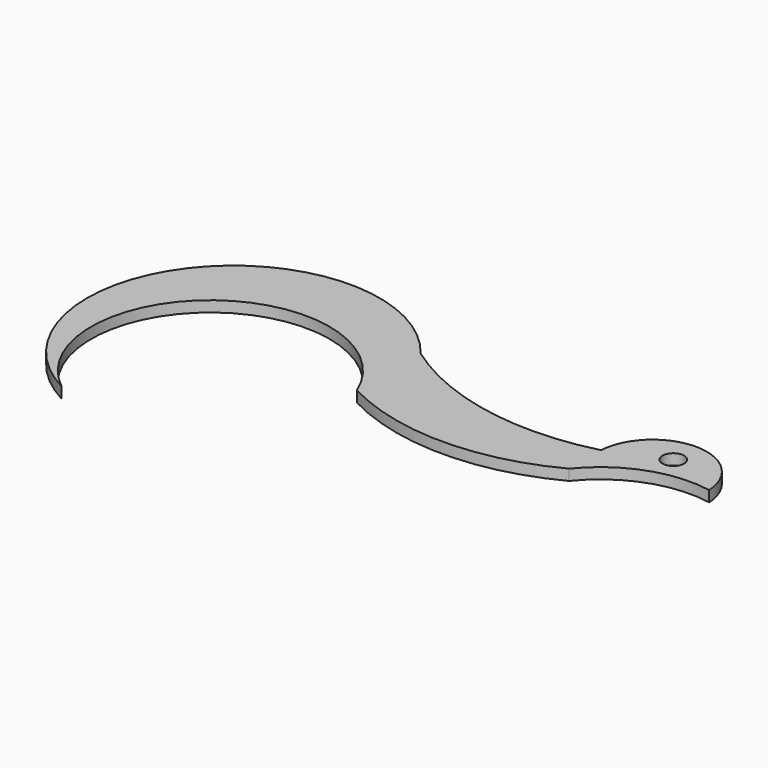
from build123d import *

# Parameters (mm, degrees)
F1_DEPTH = 5
F2_R     = 5
F3_DEPTH = 389
F4_R     = 5
F5_DEPTH = 5.001


# Not quite as in the source:
# - an extrude ends at something that could not be found from the text; its depth is read off the source's solid


with BuildPart() as f1:
    # F0 (on Top) → F1 (new body)
    with BuildSketch(Plane.XY):
        with BuildLine():
            ThreePointArc((182.6944426466, 42.1886855807), (131.7434290728, 40.4795108007), (84.8448510232, 60.4657670673))
            ThreePointArc((84.8448510232, 60.4657670673), (-20.2682643936, 62.6366103984), (0, -40.5267409035))
            ThreePointArc((0, -40.5267409035), (0.8188047448, 46.5454009095), (84.8448510232, 23.7013236039))
            ThreePointArc((84.8448510232, 23.7013236039), (133.7696468349, 11.680757797), (182.6944426466, 23.7013236039))
            ThreePointArc((182.6944426466, 23.7013236039), (205.0971207079, 39.8391466865), (232.6069186924, 42.1886855807))
            ThreePointArc((232.6069186924, 42.1886855807), (207.6506806695, 65.7101106777), (182.6944426466, 42.1886855807))
        make_face()
    extrude(amount=F1_DEPTH)

    # F2 (on Top) → F3 (cut, through all)
    with BuildSketch(Plane.XY):
        with Locations((210.5412267722, 54.1418395773)):
            Circle(F2_R)
    extrude(amount=-F3_DEPTH, mode=Mode.SUBTRACT)

    # F4 (on face) → F5 (cut, through all)
    with BuildSketch(Plane.XY.offset(5)):
        with Locations((207.6506806695, 52.6958927512)):
            Circle(F4_R)
    extrude(amount=-F5_DEPTH, mode=Mode.SUBTRACT)


solid = f1.part
